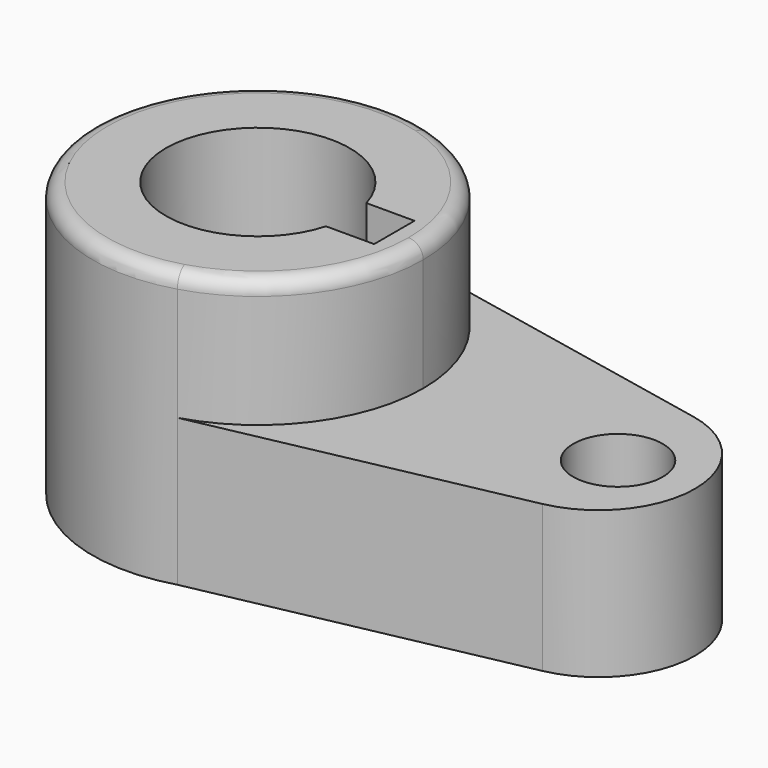
from build123d import *

# Parameters (mm, degrees)
F1_DEPTH = 25.4
F2_DEPTH = 47.498
F3_R     = 2.54


with BuildPart() as f1:
    # F0 (on Top) → F1 (new body)
    with BuildSketch(Plane.XY):
        with BuildLine():
            ThreePointArc((8.0425684433, 27.4198416814), (22.8729864498, 17.1276710579), (28.575, 0))
            ThreePointArc((28.575, 0), (22.8729864498, -17.1276710579), (8.0425684433, -27.4198416814))
            Line((8.0425684433, -27.4198416814), (62.23, -16.3154043257))
            ThreePointArc((62.23, -16.3154043257), (75.5410049965, 0), (62.23, 16.3154043257))
            Line((62.23, 16.3154043257), (8.0425684433, 27.4198416814))
        make_face()
        with BuildLine():
            ThreePointArc((69.9632073706, 0), (62.23, -7.7332073706), (54.4967926294, 0))
            ThreePointArc((54.4967926294, 0), (62.23, 7.7332073706), (69.9632073706, 0))
        make_face(mode=Mode.SUBTRACT)
    extrude(amount=F1_DEPTH)

    # F0 (on Top) → F2 (join)
    with BuildSketch(Plane.XY):
        with BuildLine():
            ThreePointArc((8.0425684433, -27.4198416814), (22.8729864498, -17.1276710579), (28.575, 0))
            ThreePointArc((28.575, 0), (22.8729864498, 17.1276710579), (8.0425684433, 27.4198416814))
            ThreePointArc((8.0425684433, 27.4198416814), (-28.575, 0), (8.0425684433, -27.4198416814))
        make_face()
        with BuildLine():
            Line((23.5818270594, 4.3561793864), (23.5818270594, 0))
            Line((23.5818270594, 0), (23.5818270594, -4.3561793864))
            Line((23.5818270594, -4.3561793864), (15.2656256391, -4.3561793864))
            ThreePointArc((15.2656256391, -4.3561793864), (-15.875, 0), (15.2656256391, 4.3561793864))
            Line((15.2656256391, 4.3561793864), (23.5818270594, 4.3561793864))
        make_face(mode=Mode.SUBTRACT)
    extrude(amount=F2_DEPTH)

    # F3
    f3_edges = [f1.edges().sort_by_distance(p)[0] for p in [
        (-8.042568, 27.419842, 47.498),
    ]]
    fillet(f3_edges, radius=F3_R)


solid = f1.part
